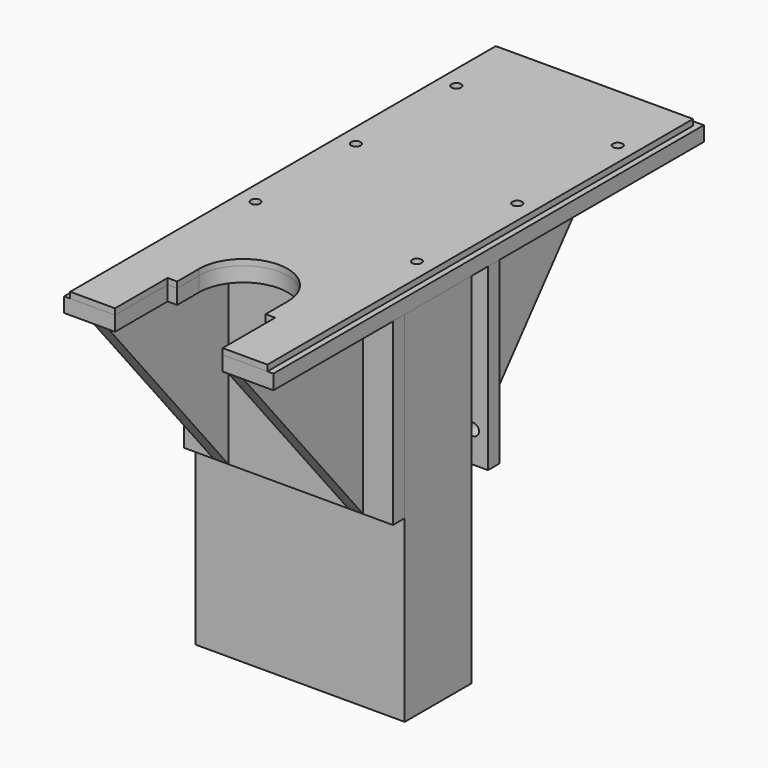
from build123d import *

# Parameters (mm, degrees)
F1_R      = 4
F2_DEPTH  = 5
F4_DEPTH  = 12.3
F5_W      = 175
F5_H      = 70
F6_DEPTH  = 300
F7_W      = 175
F7_H      = 12.3
F8_DEPTH  = 150
F11_DEPTH = 12.3
F15_R     = 5
F16_DEPTH = 12.3


# Not quite as in the source:
# - a feature of the source that left no trace in its solid (it failed there, or was rolled back) is left out


with BuildPart() as f2:
    # F1 (on Top) → F2 (new body)
    with BuildSketch(Plane.XY):
        with BuildLine():
            Line((82.5, 0), (-82.5, 0))
            Line((-82.5, 0), (-82.5, -445))
            Line((-82.5, -445), (-45, -445))
            Line((-45, -445), (-45, -390))
            Line((-45, -390), (-37, -390))
            Line((-37, -390), (-37, -367))
            ThreePointArc((-37, -367), (0, -330), (37, -367))
            Line((37, -367), (37, -390))
            Line((37, -390), (45, -390))
            Line((45, -390), (45, -445))
            Line((45, -445), (82.5, -445))
            Line((82.5, -445), (82.5, 0))
        make_face()
        with Locations((-67.5, -270)):
            Circle(F1_R, mode=Mode.SUBTRACT)
        with Locations((67.5, -270)):
            Circle(F1_R, mode=Mode.SUBTRACT)
        with Locations((-67.5, -165)):
            Circle(F1_R, mode=Mode.SUBTRACT)
        with Locations((-67.5, -60)):
            Circle(F1_R, mode=Mode.SUBTRACT)
        with Locations((67.5, -165)):
            Circle(F1_R, mode=Mode.SUBTRACT)
        with Locations((67.5, -60)):
            Circle(F1_R, mode=Mode.SUBTRACT)
    extrude(amount=F2_DEPTH)


with BuildPart() as f4:
    # F3 (on face) → F4 (new body)
    with BuildSketch(Plane(origin=(0, 0, 0), x_dir=(1, 0, 0), z_dir=(0, 0, -1))):
        with BuildLine():
            Line((-87.5, 445), (-87.5, -5))
            Line((-87.5, -5), (87.5, -5))
            Line((87.5, -5), (87.5, 445))
            Line((87.5, 445), (45, 445))
            Line((45, 445), (45, 390))
            Line((45, 390), (37, 390))
            Line((37, 390), (37, 367))
            ThreePointArc((37, 367), (0, 330), (-37, 367))
            Line((-37, 367), (-37, 390))
            Line((-37, 390), (-45, 390))
            Line((-45, 390), (-45, 445))
            Line((-45, 445), (-87.5, 445))
        make_face()
    extrude(amount=F4_DEPTH)


with BuildPart() as f6:
    # F5 (on face) → F6 (new body)
    with BuildSketch(Plane(origin=(0, 0, -12.3), x_dir=(1, 0, 0), z_dir=(0, 0, -1))):
        with Locations((0, 272.7)):
            Rectangle(F5_W, F5_H)
    extrude(amount=F6_DEPTH)


with BuildPart() as f8:
    # F7 (on face) → F8 (new body)
    with BuildSketch(Plane(origin=(0, 0, -12.3), x_dir=(1, 0, 0), z_dir=(0, 0, -1))):
        with Locations((0, 313.85)):
            Rectangle(F7_W, F7_H)
    extrude(amount=F8_DEPTH)


with BuildPart() as f8b:
    # F7 (on face) → F8, piece 2 (new body)
    with BuildSketch(Plane(origin=(0, 0, -12.3), x_dir=(1, 0, 0), z_dir=(0, 0, -1))):
        with Locations((0, 214.55)):
            Rectangle(F7_W, F7_H)
    extrude(amount=F8_DEPTH)

    # F15 (on face) → F16 (cut, through all)
    with BuildSketch(Plane(origin=(0, -208.4, 0), x_dir=(-1, 0, 0), z_dir=(0, 1, 0))):
        with Locations((75, -136.3)):
            Circle(F15_R)
        with Locations((-75, -136.3)):
            Circle(F15_R)
    extrude(amount=-F16_DEPTH, mode=Mode.SUBTRACT)


with BuildPart() as f11:
    # F10 (on offset) → F11 (new body)
    with BuildSketch(Plane(origin=(-62.5, 0, 0), x_dir=(0, -1, 0), z_dir=(-1, 0, 0))):
        Polygon((320, -162.3), (445, -12.3), (320, -12.3), align=None)
    extrude(amount=-F11_DEPTH)


with BuildPart() as f11b:
    # F10 (on offset) → F11, piece 2 (new body)
    with BuildSketch(Plane(origin=(-62.5, 0, 0), x_dir=(0, -1, 0), z_dir=(-1, 0, 0))):
        Polygon((83.4, -12.3), (208.4, -162.3), (208.4, -12.3), align=None)
    extrude(amount=-F11_DEPTH)


with BuildPart() as f12_1:
    # F12: instance of F11b
    add(f11b.part.mirror(Plane.YZ))


with BuildPart() as f12_2:
    # F12: instance of F11
    add(f11.part.mirror(Plane.YZ))


solid = Compound([f2.part, f4.part, f6.part, f8.part, f8b.part, f11.part, f11b.part, f12_1.part, f12_2.part])
